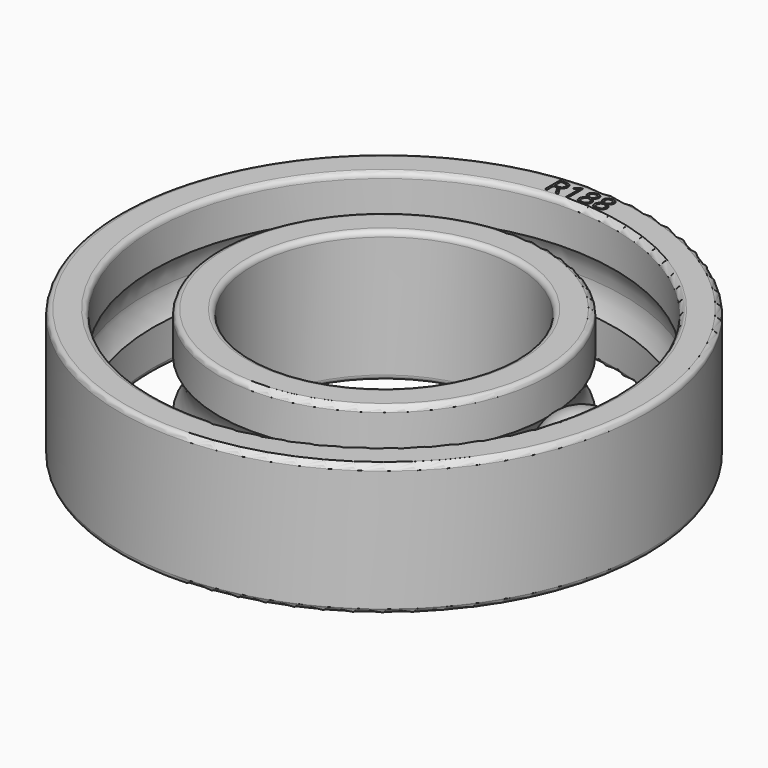
from build123d import *

# Parameters (mm, degrees)
F0_R         = 6.35
F0_R_2       = 5.55625
F2_DEPTH     = 1.5875
F1_R         = 3.96875
F1_R_2       = 3.175
F3_DEPTH     = 1.5875
F4_R         = 0.127
F4_2_R       = 0.127
F5_R         = 0.99949
F9_TEXT_SIZE = 0.6428016833
F10_DEPTH    = 0.0508


# Not quite as in the source:
# - Text() gives the source's letters only with a copy of the font that has no kerning and outlines rounded to 1/6400 em; it was checked with that copy


with BuildPart() as f2:
    # F0 (on Top) → F2 (new body, symmetric)
    with BuildSketch(Plane.XY):
        Circle(F0_R)
        Circle(F0_R_2, mode=Mode.SUBTRACT)
    extrude(amount=F2_DEPTH, both=True)

    # F4
    f4_edges = [f2.edges().sort_by_distance(p)[0] for p in [
        (-6.35, 0, 1.5875),
        (-6.35, 0, -1.5875),
        (-5.55625, 0, 1.5875),
        (-5.55625, 0, -1.5875),
    ]]
    fillet(f4_edges, radius=F4_R)


with BuildPart() as f3:
    # F1 (on Top) → F3 (new body, symmetric)
    with BuildSketch(Plane.XY):
        Circle(F1_R)
        Circle(F1_R_2, mode=Mode.SUBTRACT)
    extrude(amount=F3_DEPTH, both=True)

    # F4#2
    f4_2_edges = [f3.edges().sort_by_distance(p)[0] for p in [
        (-3.175, 0, 1.5875),
        (-3.175, 0, -1.5875),
        (-3.96875, 0, 1.5875),
        (-3.96875, 0, -1.5875),
    ]]
    fillet(f4_2_edges, radius=F4_2_R)


with BuildPart() as f6_tool:
    # F5 (on Front) → F6 (revolve)
    with BuildSketch(Plane.XZ):
        with Locations((4.7625, 0)):
            Circle(F5_R)
    revolve(axis=Axis((0, 0, 0), (0, 0, 1)))


with BuildPart() as f2_1:
    add(f2.part)

    # F6: cut by f6_tool
    add(f6_tool.part, mode=Mode.SUBTRACT)

    # F9 (on face) → F10 (cut)
    with BuildSketch(Plane.XY.offset(1.5875)):
        with Locations((-0.7541369436, 5.6971505309)):
            Text('R188', F9_TEXT_SIZE, font='Open Sans', text_align=(TextAlign.LEFT, TextAlign.BOTTOM))
    extrude(amount=-F10_DEPTH, mode=Mode.SUBTRACT)


with BuildPart() as f3_1:
    add(f3.part)

    # F6: cut by f6_tool
    add(f6_tool.part, mode=Mode.SUBTRACT)


with BuildPart() as f8:
    # F7 (on Top) → F8 (revolve)
    with BuildSketch(Plane.XY):
        with BuildLine():
            Line((4.7625, 0.99949), (4.7625, -0.99949))
            ThreePointArc((4.7625, -0.99949), (5.76199, 0), (4.7625, 0.99949))
        make_face()
    revolve(axis=Axis((4.7625, 0, 0), (0, -1, 0)))


solid = Compound([f2_1.part, f3_1.part, f8.part])
